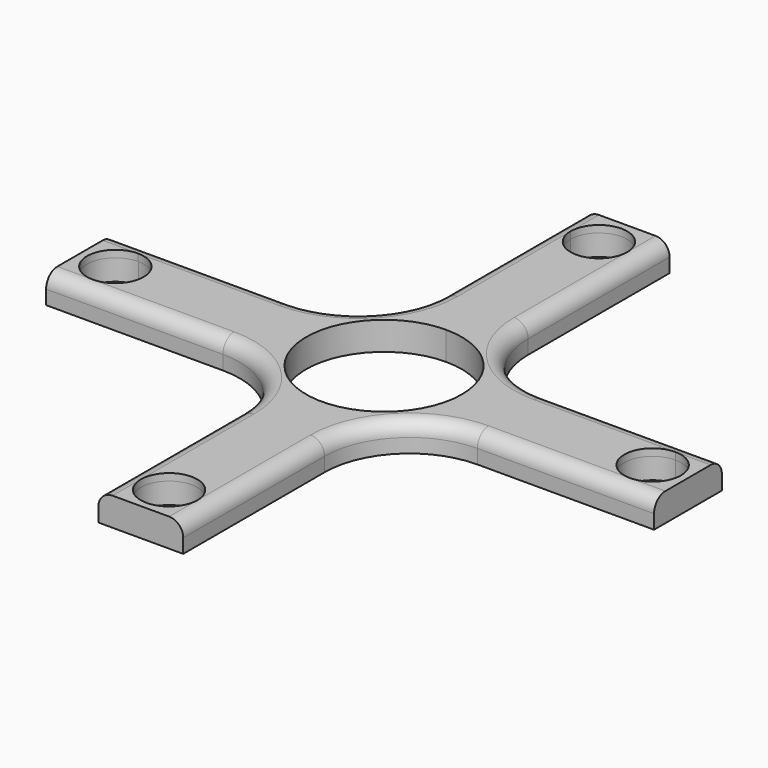
from build123d import *

# Parameters (mm, degrees)
F1_DEPTH = 4
F2_DEPTH = 3
F3_R     = 1.99999


# Not quite as in the source:
# - a fillet or chamfer is up to 0.001 mm smaller than in the source, because OpenCascade refuses the exact size
# - a feature names something its author has since deleted; it is built from what else it names


with BuildPart() as f1:
    # F0 (on Top) → F1 (new body)
    with BuildSketch(Plane.XY):
        with BuildLine():
            ThreePointArc((-4.05, 38), (0, 42.05), (4.05, 38))
            Line((4.05, 38), (6, 38))
            Line((6, 38), (6, 43))
            Line((6, 43), (-6, 43))
            Line((-6, 43), (-6, 38))
            Line((-6, 38), (-4.05, 38))
        make_face()
        with BuildLine():
            Line((6, 38), (4.05, 38))
            ThreePointArc((4.05, 38), (2.8637824638, 35.1362175362), (0, 33.95))
            ThreePointArc((0, 33.95), (-2.8637824638, 35.1362175362), (-4.05, 38))
            Line((-4.05, 38), (-6, 38))
            Line((-6, 38), (-6, 18))
            ThreePointArc((-6, 18), (-9.5147186258, 9.5147186258), (-18, 6))
            Line((-18, 6), (-38, 6))
            Line((-38, 6), (-38, 4.05))
            ThreePointArc((-38, 4.05), (-35.1362175362, 2.8637824638), (-33.95, 0))
            ThreePointArc((-33.95, 0), (-35.1362175362, -2.8637824638), (-38, -4.05))
            Line((-38, -4.05), (-38, -6))
            Line((-38, -6), (-18, -6))
            ThreePointArc((-18, -6), (-9.5147186258, -9.5147186258), (-6, -18))
            Line((-6, -18), (-6, -38))
            Line((-6, -38), (-4.05, -38))
            ThreePointArc((-4.05, -38), (0, -33.95), (4.05, -38))
            Line((4.05, -38), (6, -38))
            Line((6, -38), (6, -18))
            ThreePointArc((6, -18), (9.5147186258, -9.5147186258), (18, -6))
            Line((18, -6), (38, -6))
            Line((38, -6), (38, -4.05))
            ThreePointArc((38, -4.05), (33.95, 0), (38, 4.05))
            Line((38, 4.05), (38, 6))
            Line((38, 6), (18, 6))
            ThreePointArc((18, 6), (9.5147186258, 9.5147186258), (6, 18))
            Line((6, 18), (6, 38))
        make_face()
        with BuildLine():
            ThreePointArc((11, 0), (-7.7781745931, -7.7781745931), (0, 11))
            ThreePointArc((0, 11), (7.7781745931, 7.7781745931), (11, 0))
        make_face(mode=Mode.SUBTRACT)
        with BuildLine():
            Line((43, 6), (38, 6))
            Line((38, 6), (38, 4.05))
            ThreePointArc((38, 4.05), (40.8637824638, 2.8637824638), (42.05, 0))
            ThreePointArc((42.05, 0), (40.8637824638, -2.8637824638), (38, -4.05))
            Line((38, -4.05), (38, -6))
            Line((38, -6), (43, -6))
            Line((43, -6), (43, 6))
        make_face()
        with BuildLine():
            Line((6, -43), (6, -38))
            Line((6, -38), (4.05, -38))
            ThreePointArc((4.05, -38), (0, -42.05), (-4.05, -38))
            Line((-4.05, -38), (-6, -38))
            Line((-6, -38), (-6, -43))
            Line((-6, -43), (6, -43))
        make_face()
        with BuildLine():
            Line((-38, 4.05), (-38, 6))
            Line((-38, 6), (-43, 6))
            Line((-43, 6), (-43, -6))
            Line((-43, -6), (-38, -6))
            Line((-38, -6), (-38, -4.05))
            ThreePointArc((-38, -4.05), (-42.05, 0), (-38, 4.05))
        make_face()
        with BuildLine():
            Line((38, 4), (38, 4.05))
            ThreePointArc((38, 4.05), (33.95, 0), (38, -4.05))
            Line((38, -4.05), (38, -4))
            ThreePointArc((38, -4), (34, 0), (38, 4))
        make_face()
        with BuildLine():
            ThreePointArc((42.05, 0), (40.8637824638, 2.8637824638), (38, 4.05))
            Line((38, 4.05), (38, 4))
            ThreePointArc((38, 4), (40.8284271247, 2.8284271247), (42, 0))
            ThreePointArc((42, 0), (40.8284271247, -2.8284271247), (38, -4))
            Line((38, -4), (38, -4.05))
            ThreePointArc((38, -4.05), (40.8637824638, -2.8637824638), (42.05, 0))
        make_face()
        with BuildLine():
            Line((0, 33.95), (0, 34))
            ThreePointArc((0, 34), (-2.8284271247, 35.1715728753), (-4, 38))
            Line((-4, 38), (-4.05, 38))
            ThreePointArc((-4.05, 38), (-2.8637824638, 35.1362175362), (0, 33.95))
        make_face()
        with BuildLine():
            ThreePointArc((-33.95, 0), (-35.1362175362, 2.8637824638), (-38, 4.05))
            Line((-38, 4.05), (-38, 4))
            ThreePointArc((-38, 4), (-35.1715728753, 2.8284271247), (-34, 0))
            ThreePointArc((-34, 0), (-35.1715728753, -2.8284271247), (-38, -4))
            Line((-38, -4), (-38, -4.05))
            ThreePointArc((-38, -4.05), (-35.1362175362, -2.8637824638), (-33.95, 0))
        make_face()
        with BuildLine():
            Line((-38, 4), (-38, 4.05))
            ThreePointArc((-38, 4.05), (-42.05, 0), (-38, -4.05))
            Line((-38, -4.05), (-38, -4))
            ThreePointArc((-38, -4), (-42, 0), (-38, 4))
        make_face()
        with BuildLine():
            ThreePointArc((-4, 38), (0, 42), (4, 38))
            Line((4, 38), (4.05, 38))
            ThreePointArc((4.05, 38), (0, 42.05), (-4.05, 38))
            Line((-4.05, 38), (-4, 38))
        make_face()
        with BuildLine():
            Line((4.05, 38), (4, 38))
            ThreePointArc((4, 38), (2.8284271247, 35.1715728753), (0, 34))
            Line((0, 34), (0, 33.95))
            ThreePointArc((0, 33.95), (2.8637824638, 35.1362175362), (4.05, 38))
        make_face()
        with BuildLine():
            Line((4, -38), (4.05, -38))
            ThreePointArc((4.05, -38), (0, -33.95), (-4.05, -38))
            Line((-4.05, -38), (-4, -38))
            ThreePointArc((-4, -38), (0, -34), (4, -38))
        make_face()
        with BuildLine():
            ThreePointArc((-4.05, -38), (0, -42.05), (4.05, -38))
            Line((4.05, -38), (4, -38))
            ThreePointArc((4, -38), (0, -42), (-4, -38))
            Line((-4, -38), (-4.05, -38))
        make_face()
    extrude(amount=F1_DEPTH)

    # F0 (on Top) → F2 (cut)
    with BuildSketch(Plane.XY):
        with BuildLine():
            ThreePointArc((-4.05, -38), (0, -42.05), (4.05, -38))
            Line((4.05, -38), (4, -38))
            ThreePointArc((4, -38), (0, -42), (-4, -38))
            Line((-4, -38), (-4.05, -38))
        make_face()
        with BuildLine():
            Line((4, -38), (4.05, -38))
            ThreePointArc((4.05, -38), (0, -33.95), (-4.05, -38))
            Line((-4.05, -38), (-4, -38))
            ThreePointArc((-4, -38), (0, -34), (4, -38))
        make_face()
        with BuildLine():
            ThreePointArc((42.05, 0), (40.8637824638, 2.8637824638), (38, 4.05))
            Line((38, 4.05), (38, 4))
            ThreePointArc((38, 4), (40.8284271247, 2.8284271247), (42, 0))
            ThreePointArc((42, 0), (40.8284271247, -2.8284271247), (38, -4))
            Line((38, -4), (38, -4.05))
            ThreePointArc((38, -4.05), (40.8637824638, -2.8637824638), (42.05, 0))
        make_face()
        with BuildLine():
            ThreePointArc((42, 0), (40.8284271247, 2.8284271247), (38, 4))
            Line((38, 4), (38, 0))
            Line((38, 0), (38, -4))
            ThreePointArc((38, -4), (40.8284271247, -2.8284271247), (42, 0))
        make_face()
        with BuildLine():
            Line((38, 4), (38, 4.05))
            ThreePointArc((38, 4.05), (33.95, 0), (38, -4.05))
            Line((38, -4.05), (38, -4))
            ThreePointArc((38, -4), (34, 0), (38, 4))
        make_face()
        with BuildLine():
            Line((38, 0), (38, 4))
            ThreePointArc((38, 4), (34, 0), (38, -4))
            Line((38, -4), (38, 0))
        make_face()
        with BuildLine():
            ThreePointArc((-4, 38), (0, 42), (4, 38))
            Line((4, 38), (4.05, 38))
            ThreePointArc((4.05, 38), (0, 42.05), (-4.05, 38))
            Line((-4.05, 38), (-4, 38))
        make_face()
        with BuildLine():
            Line((4.05, 38), (4, 38))
            ThreePointArc((4, 38), (2.8284271247, 35.1715728753), (0, 34))
            Line((0, 34), (0, 33.95))
            ThreePointArc((0, 33.95), (2.8637824638, 35.1362175362), (4.05, 38))
        make_face()
        with BuildLine():
            Line((0, 33.95), (0, 34))
            ThreePointArc((0, 34), (-2.8284271247, 35.1715728753), (-4, 38))
            Line((-4, 38), (-4.05, 38))
            ThreePointArc((-4.05, 38), (-2.8637824638, 35.1362175362), (0, 33.95))
        make_face()
        with BuildLine():
            Line((0, 34), (0, 38))
            Line((0, 38), (-4, 38))
            ThreePointArc((-4, 38), (-2.8284271247, 35.1715728753), (0, 34))
        make_face()
        with BuildLine():
            Line((-38, 4), (-38, 4.05))
            ThreePointArc((-38, 4.05), (-42.05, 0), (-38, -4.05))
            Line((-38, -4.05), (-38, -4))
            ThreePointArc((-38, -4), (-42, 0), (-38, 4))
        make_face()
        with BuildLine():
            ThreePointArc((-33.95, 0), (-35.1362175362, 2.8637824638), (-38, 4.05))
            Line((-38, 4.05), (-38, 4))
            ThreePointArc((-38, 4), (-35.1715728753, 2.8284271247), (-34, 0))
            ThreePointArc((-34, 0), (-35.1715728753, -2.8284271247), (-38, -4))
            Line((-38, -4), (-38, -4.05))
            ThreePointArc((-38, -4.05), (-35.1362175362, -2.8637824638), (-33.95, 0))
        make_face()
    extrude(amount=F2_DEPTH, mode=Mode.SUBTRACT)

    # F3 (radius 2 in the source; OpenCascade refuses exactly that, so slightly less here)
    f3_edges = [f1.edges().sort_by_distance(p)[0] for p in [
        (-6, 30.5, 4),
        (6, 30.5, 4),
        (30.5, -6, 4),
        (9.514719, -9.514719, 4),
        (-9.514719, -9.514719, 4),
    ]]
    fillet(f3_edges, radius=F3_R)


solid = f1.part
